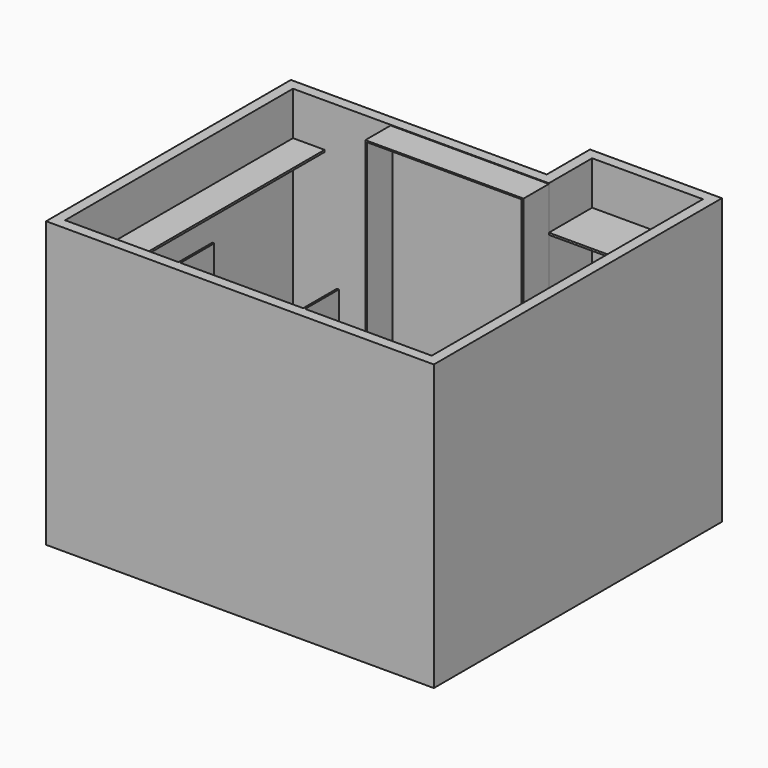
from build123d import *

# Parameters (mm, degrees)
F1_DEPTH  = 2743.2
F2_W      = 762
F2_H      = 1524
F3_DEPTH  = 558.8
F4_W      = 1524
F4_H      = 2730.5
F4_W_2    = 1485.9
F4_H_2    = 2705.1
F5_DEPTH  = 304.8
F6_W      = 1219.2
F6_H      = 19.05
F7_DEPTH  = 406.4
F8_W      = 1219.2
F8_H      = 1219.2
F9_DEPTH  = 609.6
F10_W     = 19.05
F10_H     = 406.4
F11_DEPTH = 1524
F12_W     = 3124.2
F12_H     = 19.05
F13_DEPTH = 406.4
F14_W     = 2857.5
F14_H     = 19.05
F15_DEPTH = 406.4
F16_W     = 3530.6
F16_H     = 19.05
F17_DEPTH = 3263.9
F18_W     = 2921
F18_H     = 2438.4
F19_DEPTH = 19.05
F20_W     = 2362.2
F20_H     = 419.1000000008
F21_DEPTH = 2324.101


with BuildPart() as f1:
    # F0 (on Top) → F1 (new body)
    with BuildSketch(Plane.XY):
        Polygon((2362.2, 3365.5), (2362.2, 2844.8), (-101.6, 2844.8), (-101.6, -101.6), (3632.2, -101.6), (3632.2, 3365.5), align=None)
        Polygon((3530.6, 0), (0, 0), (0, 2743.2), (2463.8, 2743.2), (2463.8, 3263.9), (3530.6, 3263.9), align=None, mode=Mode.SUBTRACT)
    extrude(amount=F1_DEPTH)

    # F2 (on face) → F3 (join)
    with BuildSketch(Plane.XZ.offset(-3263.9)):
        with Locations((2857.5, 762)):
            Rectangle(F2_W, F2_H)
    extrude(amount=F3_DEPTH)

    # F6 (on face) → F7 (join)
    with BuildSketch(Plane.YZ):
        with Locations((609.6, 1838.325)):
            Rectangle(F6_W, F6_H)
    extrude(amount=F7_DEPTH)

    # F8 (on face) → F9 (join)
    with BuildSketch(Plane(origin=(0, 0, 0), x_dir=(-1, 0, 0), z_dir=(0, 1, 0))):
        with Locations((-1701.8, 609.6)):
            Rectangle(F8_W, F8_H)
    extrude(amount=F9_DEPTH)

    # F10 (on face) → F11 (join)
    with BuildSketch(Plane.XY.offset(1219.2)):
        with Locations((2301.875, 203.2)):
            Rectangle(F10_W, F10_H)
        with Locations((1101.725, 203.2)):
            Rectangle(F10_W, F10_H)
    extrude(amount=F11_DEPTH)

    # F12 (on face) → F13 (join)
    with BuildSketch(Plane(origin=(0, 0, 0), x_dir=(-1, 0, 0), z_dir=(0, 1, 0))):
        with Locations((-1968.5, 1838.325)):
            Rectangle(F12_W, F12_H)
    extrude(amount=F13_DEPTH)

    # F14 (on face) → F15 (join)
    with BuildSketch(Plane(origin=(3530.6, 0, 0), x_dir=(0, -1, 0), z_dir=(-1, 0, 0))):
        with Locations((-1835.15, 1838.325)):
            Rectangle(F14_W, F14_H)
    extrude(amount=F15_DEPTH)

    # F16 (on face) → F17 (join, through all)
    with BuildSketch(Plane(origin=(0, 0, 0), x_dir=(-1, 0, 0), z_dir=(0, 1, 0))):
        with Locations((-1765.3, 2314.575)):
            Rectangle(F16_W, F16_H)
    extrude(amount=F17_DEPTH)

    # F18 (on face) → F19 (cut)
    with BuildSketch(Plane.XY.offset(2324.1)):
        with Locations((1765.3, 1524)):
            Rectangle(F18_W, F18_H)
    extrude(amount=-F19_DEPTH, mode=Mode.SUBTRACT)

    # F20 (on face) → F21 (cut, through all)
    with BuildSketch(Plane.XY.offset(2324.1)):
        with Locations((1181.1, 3054.3500000004)):
            Rectangle(F20_W, F20_H)
    extrude(amount=-F21_DEPTH, mode=Mode.SUBTRACT)


with BuildPart() as f5:
    # F4 (on face) → F5 (new body)
    with BuildSketch(Plane.XZ.offset(-2743.2)):
        with Locations((1701.8, 1371.6)):
            Rectangle(F4_W, F4_H)
        with Locations((1701.8, 1371.6)):
            Rectangle(F4_W_2, F4_H_2, mode=Mode.SUBTRACT)
    extrude(amount=F5_DEPTH)


solid = Compound([f1.part, f5.part])
